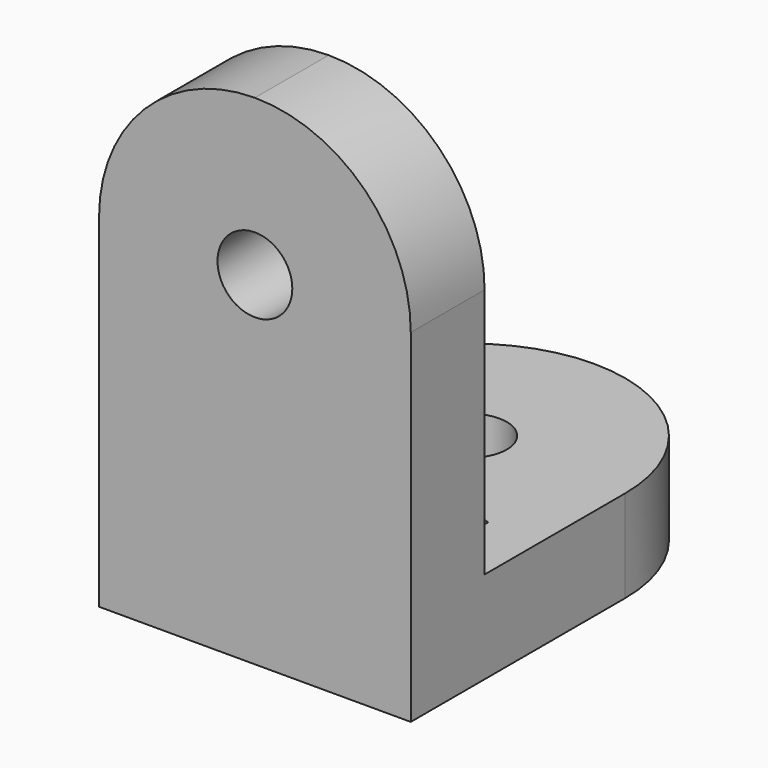
from build123d import *

# Parameters (mm, degrees)
F0_R     = 1.5
F2_DEPTH = 3.7
F1_R     = 1.5
F3_DEPTH = 3.7
F6_W     = 2
F6_H     = 4
F7_DEPTH = 4


with BuildPart() as f2:
    # F0 (on Front) → F2 (new body)
    with BuildSketch(Plane.XZ):
        with BuildLine():
            Line((0, 13.75), (0, 0))
            Line((0, 0), (12.5, 0))
            Line((12.5, 0), (12.5, 13.75))
            ThreePointArc((12.5, 13.75), (10.6694173824, 18.1694173824), (6.25, 20))
            ThreePointArc((6.25, 20), (1.8305826176, 18.1694173824), (0, 13.75))
        make_face()
        with Locations((6.25, 13.75)):
            Circle(F0_R, mode=Mode.SUBTRACT)
    extrude(amount=-F2_DEPTH)

    # F1 (on Top) → F3 (join)
    with BuildSketch(Plane.XY):
        with BuildLine():
            Line((0, 10.75), (0, 0))
            Line((0, 0), (12.5, 0))
            Line((12.5, 0), (12.5, 10.75))
            ThreePointArc((12.5, 10.75), (10.6694173824, 15.1694173824), (6.25, 17))
            ThreePointArc((6.25, 17), (1.8305826176, 15.1694173824), (0, 10.75))
        make_face()
        with Locations((6.25, 10.75)):
            Circle(F1_R, mode=Mode.SUBTRACT)
    extrude(amount=F3_DEPTH)

    # F6 (on face) → F7 (join)
    with BuildSketch(Plane(origin=(0, 5.1142135624, 5.1142135624), x_dir=(1, 0, 0), z_dir=(0, -0.7071067812, -0.7071067812))):
        with Locations((9.375, 0)):
            Rectangle(F6_W, F6_H)
        with Locations((3.125, 0)):
            Rectangle(F6_W, F6_H)
    extrude(amount=F7_DEPTH)


solid = f2.part
